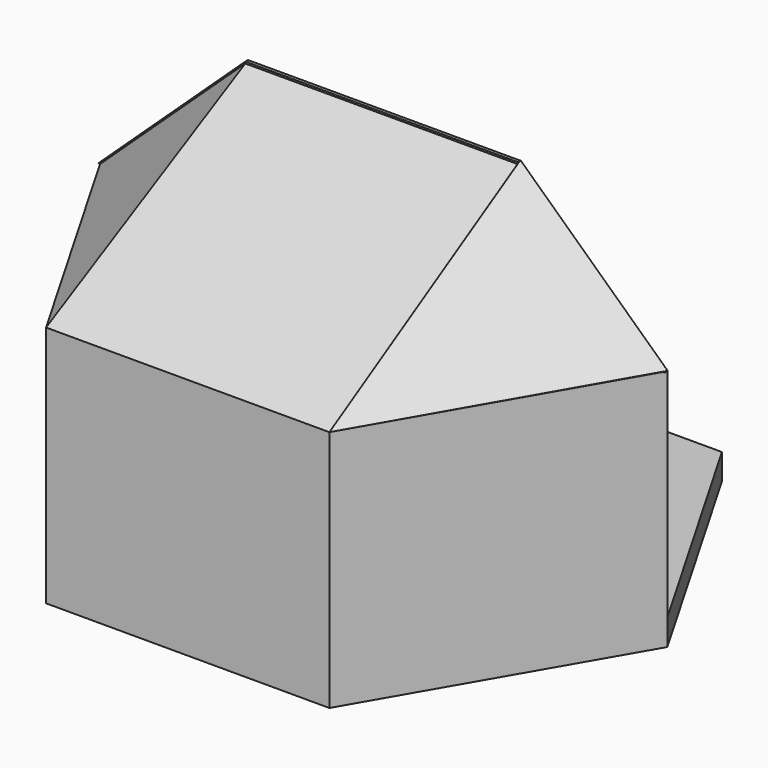
from build123d import *

# Parameters (mm, degrees)
F0_W      = 50
F0_H      = 12.5
F1_DEPTH  = 8
F2_DEPTH  = 75
F4_DEPTH  = 8
F7_DEPTH  = 3
F8_DEPTH  = 1
F11_DEPTH = 3
F14_DEPTH = 3
F15_DEPTH = 8
F16_DEPTH = 25
F17_DEPTH = 8


# Not quite as in the source:
# - a feature names something its author has since deleted; it is built from what else it names


with BuildPart() as f1:
    # F0 (on Top) → F1 (new body)
    with BuildSketch(Plane.XY):
        Polygon((-42.0179491924, 72.7772228311), (-60.5095952989, 40.7487522591), (-57.9695070384, 39.3207329262), (-55.5194165334, 43.6791064608), (-50.2642610162, 40.7248836223), (-52.7144317239, 36.366367418), (-57.615009792, 27.6494680496), (-60.0654171506, 23.2910848888), (-65.3204122546, 26.2455930623), (-62.870004896, 30.6039762231), (-65.5097997054, 32.0881441788), (-84.0358983849, 0), (-42.0179491924, -72.7772228311), (42.0179491924, -72.7772228311), (84.0358983849, 0), (42.0179491924, 72.7772228311), align=None)
        with Locations((0, 54.5829171234)):
            Rectangle(F0_W, F0_H, mode=Mode.SUBTRACT)
    extrude(amount=F1_DEPTH)

    # F0 (on Top) → F2 (join)
    with BuildSketch(Plane.XY):
        Polygon((43.75, -75.7772228311), (87.5, 0), (84.0358983849, 0), (42.0179491924, -72.7772228311), (-42.0179491924, -72.7772228311), (-84.0358983849, 0), (-87.5, 0), (-43.75, -75.7772228311), align=None)
    extrude(amount=F2_DEPTH)

    # F0 (on Top) → F4 (join)
    with BuildSketch(Plane.XY):
        Polygon((43.75, 75.7772228311), (-43.75, 75.7772228311), (-63.1248363216, 42.2190219338), (-60.5095952989, 40.7487522591), (-42.0179491924, 72.7772228311), (42.0179491924, 72.7772228311), (84.0358983849, 0), (87.5, 0), align=None)
    extrude(amount=F4_DEPTH)

    # F6 (on face) → F7 (join)
    with BuildSketch(Plane(origin=(0, -50.1312366318, 89.3836679776), x_dir=(1, 0, 0), z_dir=(0, 0.4891706574, -0.872188092))):
        Polygon((43.75, 29.4041920927), (0, 29.4041920927), (-43.75, 29.4041920927), (-42.01795, -57.4775522498), (42.01795, -57.4775522498), align=None)
    extrude(amount=F7_DEPTH)

    # F3 (on Front) → F8 (join)
    with BuildSketch(Plane.XZ):
        Polygon((-42.01795, 114.5), (0, 114.5), (42.01795, 114.5), (84.0359, 75), (87.5, 75), (42.01795, 117.5), (0, 117.5), (-42.01795, 117.5), (-87.5, 75), (-84.0359, 75), align=None)
    extrude(amount=F8_DEPTH)

    # F10 (on face) → F11 (join)
    with BuildSketch(Plane(origin=(-67.6846727043, -39.0777640058, 72.4338274863), x_dir=(0.7723629594, -0.3015876344, 0.5590173143), z_dir=(-0.6351814378, -0.3667221741, 0.6797495039))):
        Polygon((33.2314262259, 55.789645187), (-25.6554603702, 35.6104118215), (30.9888924807, -31.0804218073), align=None)
    extrude(amount=-F11_DEPTH)

    # F13 (on face) → F14 (join)
    with BuildSketch(Plane(origin=(67.6756688636, -39.5950852503, 72.4241918832), x_dir=(0.7733047167, 0.3041472681, -0.556322078), z_dir=(-0.6340345536, 0.3709553614, -0.6785221475))):
        Polygon((-30.939509805, 30.5117392321), (-32.8751652468, -56.3649154418), (25.9400068576, -35.9776056011), align=None)
    extrude(amount=F14_DEPTH)

    # F0 (on Top) → F15 (join)
    with BuildSketch(Plane.XY):
        with Locations((0, 54.5829171234)):
            Rectangle(F0_W, F0_H)
    extrude(amount=F15_DEPTH)

    # F0 (on Top) → F16 (cut)
    with BuildSketch(Plane.XY):
        Polygon((-57.9695070384, 39.3207329262), (-60.5095952989, 40.7487522591), (-65.5097997054, 32.0881441788), (-62.870004896, 30.6039762231), (-57.615009792, 27.6494680496), (-52.7144317239, 36.366367418), align=None)
    extrude(amount=-F16_DEPTH, mode=Mode.SUBTRACT)

    # F0 (on Top) → F17 (join)
    with BuildSketch(Plane.XY):
        Polygon((-65.5097997054, 32.0881441788), (-68.125, 33.5584843966), (-87.5, 0), (-84.0358983849, 0), align=None)
    extrude(amount=F17_DEPTH)


solid = f1.part
